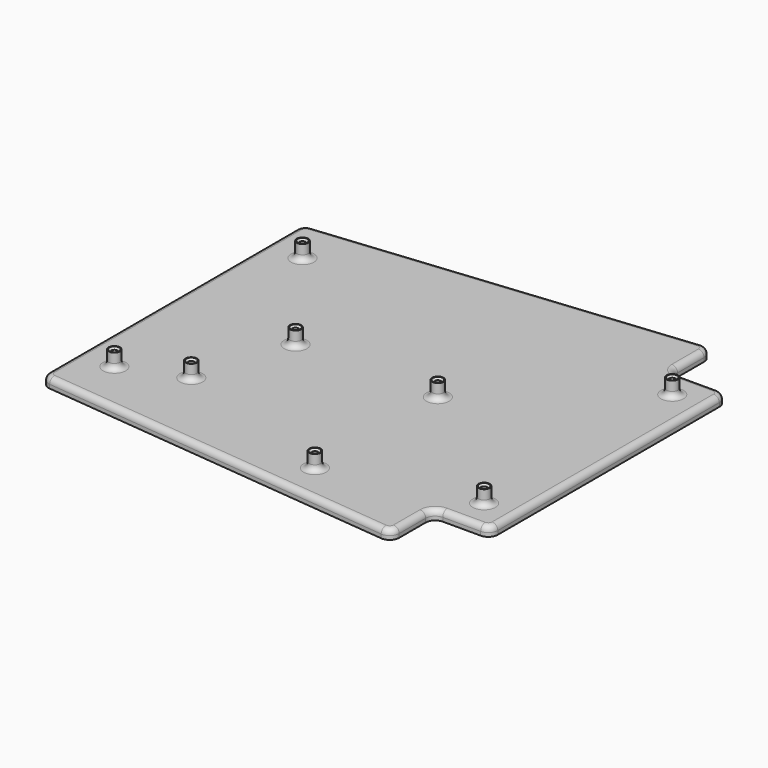
from build123d import *

# Parameters (mm, degrees)
F0_R     = 1.5
F1_DEPTH = 2.5
F2_R     = 2.5
F3_R     = 1.5
F0_R_2   = 0.8
F4_DEPTH = 6.5
F5_R     = 1.5
F6_SIZE  = 0.5


# Not quite as in the source:
# - a feature names something its author has since deleted; it is built from what else it names


with BuildPart() as f1:
    # F0 (on Top) → F1 (new body)
    with BuildSketch(Plane.XY):
        Polygon((115, 39), (100, 39), (100, 53), (0, 43), (0, -43), (100, -53), (100, -39), (115, -39), align=None)
        with Locations((9.523, -31)):
            Circle(F0_R, mode=Mode.SUBTRACT)
        with Locations((25, -25)):
            Circle(F0_R, mode=Mode.SUBTRACT)
        with Locations((70, -40.5)):
            Circle(F0_R, mode=Mode.SUBTRACT)
        with Locations((107, -31)):
            Circle(F0_R, mode=Mode.SUBTRACT)
        with Locations((32.483, 0)):
            Circle(F0_R, mode=Mode.SUBTRACT)
        with Locations((9.523, 31)):
            Circle(F0_R, mode=Mode.SUBTRACT)
        with Locations((70, 0)):
            Circle(F0_R, mode=Mode.SUBTRACT)
        with Locations((107, 31)):
            Circle(F0_R, mode=Mode.SUBTRACT)
    extrude(amount=F1_DEPTH)

    # F2
    f2_edges = [f1.edges().sort_by_distance(p)[0] for p in [
        (100, 39, 1.25),
        (100, 53, 1.25),
        (115, 39, 1.25),
        (0, 43, 1.25),
        (115, -39, 1.25),
        (100, -39, 1.25),
        (100, -53, 1.25),
        (0, -43, 1.25),
    ]]
    fillet(f2_edges, radius=F2_R)

    # F3
    f3_edges = [f1.edges().sort_by_distance(p)[0] for p in [
        (0, 0, 2.5),
        (115, 0, 2.5),
        (49.751241, 47.975124, 2.5),
        (49.751241, -47.975124, 2.5),
        (100, -45.868766, 2.5),
        (107.5, -39, 2.5),
        (107.5, 39, 2.5),
        (100, 45.868766, 2.5),
    ]]
    fillet(f3_edges, radius=F3_R)

    # F0 (on Top) → F4 (join)
    with BuildSketch(Plane.XY):
        with Locations((107, 31)):
            Circle(F0_R)
        with Locations((107, 31)):
            Circle(F0_R_2, mode=Mode.SUBTRACT)
        with Locations((70, 0)):
            Circle(F0_R)
        with Locations((70, 0)):
            Circle(F0_R_2, mode=Mode.SUBTRACT)
        with Locations((107, -31)):
            Circle(F0_R)
        with Locations((107, -31)):
            Circle(F0_R_2, mode=Mode.SUBTRACT)
        with Locations((70, -40.5)):
            Circle(F0_R)
        with Locations((70, -40.5)):
            Circle(F0_R_2, mode=Mode.SUBTRACT)
        with Locations((25, -25)):
            Circle(F0_R)
        with Locations((25, -25)):
            Circle(F0_R_2, mode=Mode.SUBTRACT)
        with Locations((9.523, -31)):
            Circle(F0_R)
        with Locations((9.523, -31)):
            Circle(F0_R_2, mode=Mode.SUBTRACT)
        with Locations((9.523, 31)):
            Circle(F0_R)
        with Locations((9.523, 31)):
            Circle(F0_R_2, mode=Mode.SUBTRACT)
        with Locations((32.483, 0)):
            Circle(F0_R)
        with Locations((32.483, 0)):
            Circle(F0_R_2, mode=Mode.SUBTRACT)
    extrude(amount=F4_DEPTH)

    # F5
    f5_edges = [f1.edges().sort_by_distance(p)[0] for p in [
        (68.5, 0, 2.5),
        (23.5, -25, 2.5),
        (8.023, -31, 2.5),
        (8.023, 31, 2.5),
        (68.5, -40.5, 2.5),
        (105.5, -31, 2.5),
        (105.5, 31, 2.5),
        (30.983, 0, 2.5),
    ]]
    fillet(f5_edges, radius=F5_R)

    # F6
    f6_edges = [f1.edges().sort_by_distance(p)[0] for p in [
        (106.2, 31, 6.5),
        (106.2, -31, 6.5),
        (69.2, -40.5, 6.5),
        (69.2, 0, 6.5),
        (8.723, 31, 6.5),
        (24.2, -25, 6.5),
        (8.723, -31, 6.5),
        (31.683, 0, 6.5),
    ]]
    chamfer(f6_edges, length=F6_SIZE)


solid = f1.part
